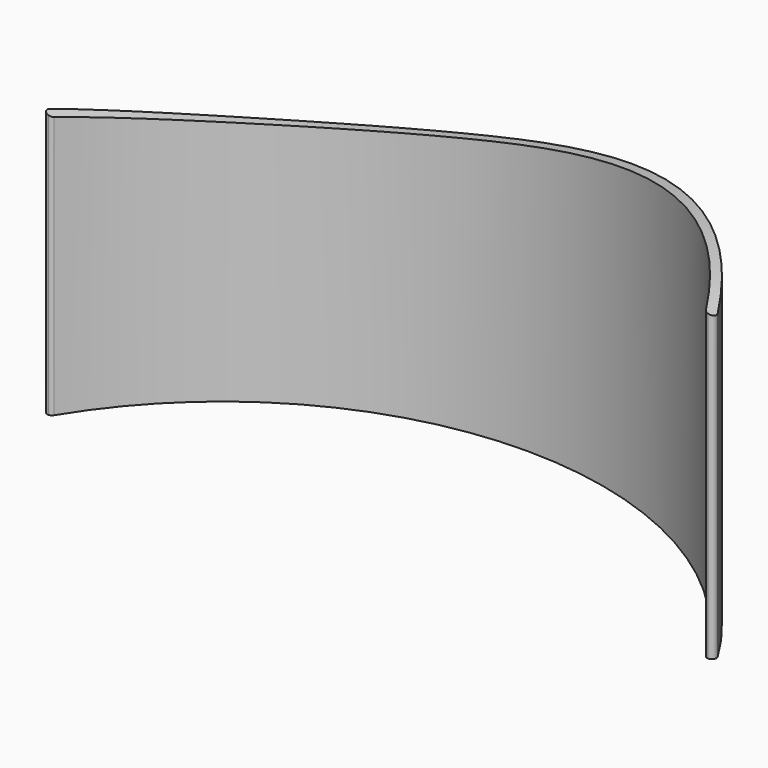
from build123d import *

# Parameters (mm, degrees)
F1_DEPTH = 350
F2_R     = 4.99999
F5_DEPTH = 445.001


# Not quite as in the source:
# - a fillet or chamfer is up to 0.001 mm smaller than in the source, because OpenCascade refuses the exact size


with BuildPart() as f1:
    # F0 (on Top) → F1 (new body)
    with BuildSketch(Plane.XY):
        with BuildLine():
            ThreePointArc((-352.143192, 209.988505), (0, 410), (352.143192, 209.988505))
            Line((352.143192, 209.988505), (363.737306, 209.988505))
            ThreePointArc((363.737306, 209.988505), (0, 420), (-363.737306, 209.988505))
            Line((-363.737306, 209.988505), (-352.143192, 209.988505))
        make_face()
    extrude(amount=F1_DEPTH)

    # F2 (radius 5 in the source; OpenCascade refuses exactly that, so slightly less here)
    f2_edges = [f1.edges().sort_by_distance(p)[0] for p in [
        (-352.143192, 209.988505, 175),
        (-363.737306, 209.988505, 175),
        (352.143192, 209.988505, 175),
        (363.737306, 209.988505, 175),
    ]]
    fillet(f2_edges, radius=F2_R)

    # F4 (on offset) → F5 (cut, through all)
    with BuildSketch(Plane.XZ.offset(25)):
        with BuildLine():
            Line((-435.187875, 462.972403), (-435.187875, 317.413754))
            add(Edge.make_bspline(
                [(-435.187875, 317.413754), (-412.820875, 308.514677), (-319.839202, 258.096258), (-61.092997, 258.830108), (356.413959, 382.935619), (417.542687, 277.268735), (422.748376, 267.598979)],
                knots=[0, 0, 0, 0, 0.174054, 0.451516, 0.791762, 0.935723, 0.935723, 0.935723, 0.935723], degree=3))
            Line((422.748376, 267.598979), (416.810036, 462.972403))
            Line((416.810036, 462.972403), (-435.187875, 462.972403))
        make_face()
    extrude(amount=-F5_DEPTH, mode=Mode.SUBTRACT)


solid = f1.part
